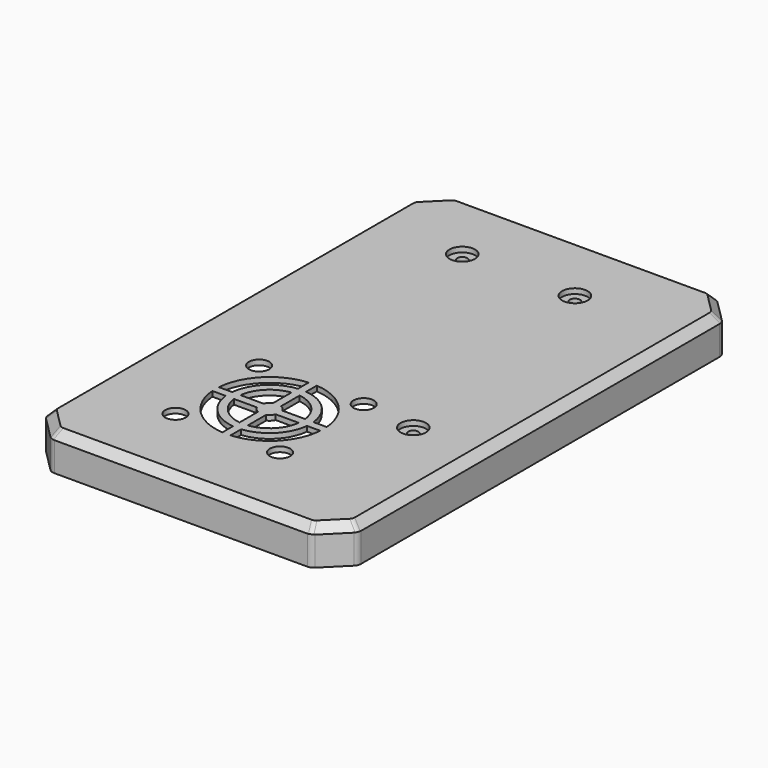
from build123d import *

# Parameters (mm, degrees)
F3_DEPTH  = 1.5875
F1_R      = 5.08
F1_R_2    = 1.5875
F4_DEPTH  = 10
F5_DEPTH  = 10
F6_R      = 3.96875
F7_DEPTH  = 1.5875
F8_R      = 3.175
F9_DEPTH  = 11.5885
F10_SIZE  = 2.54
F11_F1_R  = 2.54
F11_F2_R  = 2.54
F11_F3_R  = 2.54
F11_F4_R  = 2.54
F11_F5_R  = 2.54
F11_F6_R  = 2.54
F11_F7_R  = 2.54
F11_F8_R  = 2.54
F11_F9_R  = 2.54
F11_F10_R = 2.54
F11_F11_R = 2.54
F11_F12_R = 2.54
F11_F13_R = 2.54
F11_F14_R = 2.54
F11_F15_R = 2.54
F11_F16_R = 2.54


with BuildPart() as f3:
    # F0 (on Top) → F3 (new body)
    with BuildSketch(Plane.XY):
        Polygon((-40.4276280605, 79.0125), (-48.6375, 70.8026280605), (-48.6375, -70.8026280605), (-40.4276280605, -79.0125), (40.4276280605, -79.0125), (48.6375, -70.8026280605), (48.6375, 70.8026280605), (40.4276280605, 79.0125), align=None)
        Polygon((-45.4625, 69.4875), (-39.1125, 75.8375), (39.1125, 75.8375), (45.4625, 69.4875), (45.4625, -69.4875), (39.1125, -75.8375), (-39.1125, -75.8375), (-45.4625, -69.4875), align=None, mode=Mode.SUBTRACT)
        Polygon((39.1125, 75.8375), (-39.1125, 75.8375), (-45.4625, 69.4875), (-45.4625, -69.4875), (-39.1125, -75.8375), (39.1125, -75.8375), (45.4625, -69.4875), (45.4625, 69.4875), align=None)
    extrude(amount=F3_DEPTH)

    # F1 (on Top) → F4 (join)
    with BuildSketch(Plane.XY):
        with Locations((27.6825, -23.2224922)):
            Circle(F1_R)
        with Locations((27.6825, -23.2224922)):
            Circle(F1_R_2, mode=Mode.SUBTRACT)
        with Locations((14.9825, 55.5175)):
            Circle(F1_R)
        with Locations((14.9825, 55.5175)):
            Circle(F1_R_2, mode=Mode.SUBTRACT)
        with Locations((-20.0625, 55.5175)):
            Circle(F1_R)
        with Locations((-20.0625, 55.5175)):
            Circle(F1_R_2, mode=Mode.SUBTRACT)
    extrude(amount=-F4_DEPTH)

    # F0 (on Top) → F5 (join)
    with BuildSketch(Plane.XY):
        Polygon((-40.4276280605, 79.0125), (-48.6375, 70.8026280605), (-48.6375, -70.8026280605), (-40.4276280605, -79.0125), (40.4276280605, -79.0125), (48.6375, -70.8026280605), (48.6375, 70.8026280605), (40.4276280605, 79.0125), align=None)
        Polygon((-45.4625, 69.4875), (-39.1125, 75.8375), (39.1125, 75.8375), (45.4625, 69.4875), (45.4625, -69.4875), (39.1125, -75.8375), (-39.1125, -75.8375), (-45.4625, -69.4875), align=None, mode=Mode.SUBTRACT)
    extrude(amount=-F5_DEPTH)

    # F6 (on face) → F7 (cut)
    with BuildSketch(Plane.XY.offset(1.5875)):
        with Locations((-20.0625, 55.5175)):
            Circle(F6_R)
        with Locations((14.9825, 55.5175)):
            Circle(F6_R)
        with Locations((27.6825, -23.2224922)):
            Circle(F6_R)
    extrude(amount=-F7_DEPTH, mode=Mode.SUBTRACT)

    # F8 (on face) → F9 (cut, through all)
    with BuildSketch(Plane.XY.offset(1.5875)):
        with Locations((-22.00625, -21.06875)):
            Circle(F8_R)
        with Locations((10.5375, -21.06875)):
            Circle(F8_R)
        with Locations((10.5375, -53.6125)):
            Circle(F8_R)
        with Locations((-22.00625, -53.6125)):
            Circle(F8_R)
        with BuildLine():
            Line((-18.3707154513, -38.610625), (-22.5138820324, -38.610625))
            ThreePointArc((-22.5138820324, -38.610625), (-17.6332143604, -49.2394643604), (-7.004375, -54.1201320324))
            Line((-7.004375, -54.1201320324), (-7.004375, -49.9769654513))
            ThreePointArc((-7.004375, -49.9769654513), (-14.7146311211, -46.3208811211), (-18.3707154513, -38.610625))
        make_face()
        with BuildLine():
            ThreePointArc((-8.6443105663, -36.070625), (-7.9794390303, -35.0955609697), (-7.004375, -34.4306894337))
            Line((-7.004375, -34.4306894337), (-7.004375, -27.2603125048))
            ThreePointArc((-7.004375, -27.2603125048), (-12.9185798969, -30.1564201031), (-15.8146874952, -36.070625))
            Line((-15.8146874952, -36.070625), (-8.6443105663, -36.070625))
        make_face()
        with BuildLine():
            Line((-4.464375, -27.2603125048), (-4.464375, -34.4306894337))
            ThreePointArc((-4.464375, -34.4306894337), (-3.4893109697, -35.0955609697), (-2.8244394337, -36.070625))
            Line((-2.8244394337, -36.070625), (4.3459374952, -36.070625))
            ThreePointArc((4.3459374952, -36.070625), (1.4498298969, -30.1564201031), (-4.464375, -27.2603125048))
        make_face()
        with BuildLine():
            Line((4.3459374952, -38.610625), (-2.8244394337, -38.610625))
            ThreePointArc((-2.8244394337, -38.610625), (-3.4893109697, -39.5856890303), (-4.464375, -40.2505605663))
            Line((-4.464375, -40.2505605663), (-4.464375, -47.4209374952))
            ThreePointArc((-4.464375, -47.4209374952), (1.4498298969, -44.5248298969), (4.3459374952, -38.610625))
        make_face()
        with BuildLine():
            Line((-7.004375, -47.4209374952), (-7.004375, -40.2505605663))
            ThreePointArc((-7.004375, -40.2505605663), (-7.9794390303, -39.5856890303), (-8.6443105663, -38.610625))
            Line((-8.6443105663, -38.610625), (-15.8146874952, -38.610625))
            ThreePointArc((-15.8146874952, -38.610625), (-12.9185798969, -44.5248298969), (-7.004375, -47.4209374952))
        make_face()
        with BuildLine():
            Line((-22.5138820324, -36.070625), (-18.3707154513, -36.070625))
            ThreePointArc((-18.3707154513, -36.070625), (-14.7146311211, -28.3603688789), (-7.004375, -24.7042845487))
            Line((-7.004375, -24.7042845487), (-7.004375, -20.5611179676))
            ThreePointArc((-7.004375, -20.5611179676), (-17.6332143604, -25.4417856396), (-22.5138820324, -36.070625))
        make_face()
        with BuildLine():
            ThreePointArc((-4.464375, -24.7042845487), (3.2458811211, -28.3603688789), (6.9019654513, -36.070625))
            Line((6.9019654513, -36.070625), (11.0451320324, -36.070625))
            ThreePointArc((11.0451320324, -36.070625), (6.1644643604, -25.4417856396), (-4.464375, -20.5611179676))
            Line((-4.464375, -20.5611179676), (-4.464375, -24.7042845487))
        make_face()
        with BuildLine():
            Line((11.0451320324, -38.610625), (6.9019654513, -38.610625))
            ThreePointArc((6.9019654513, -38.610625), (3.2458811211, -46.3208811211), (-4.464375, -49.9769654513))
            Line((-4.464375, -49.9769654513), (-4.464375, -54.1201320324))
            ThreePointArc((-4.464375, -54.1201320324), (6.1644643604, -49.2394643604), (11.0451320324, -38.610625))
        make_face()
    extrude(amount=-F9_DEPTH, mode=Mode.SUBTRACT)

    # F10
    f10_edges = [f3.edges().sort_by_distance(p)[0] for p in [
        (0, 79.0125, 1.5875),
        (-44.532564, 74.907564, 1.5875),
        (-48.6375, 0, 1.5875),
        (44.532564, 74.907564, 1.5875),
        (48.6375, 0, 1.5875),
        (-44.532564, -74.907564, 1.5875),
        (0, -79.0125, 1.5875),
        (44.532564, -74.907564, 1.5875),
    ]]
    chamfer(f10_edges, length=F10_SIZE)

    # F11: fillet of radius 2.54 on 16 edges, made by hand

    # F11_f1
    f11_f1_edges = [f3.edges().sort_by_distance(p)[0] for p in [
        (-40.4276280605, 79.0125, -5.47625),
    ]]
    fillet(f11_f1_edges, radius=F11_F1_R)

    # F11_f2
    f11_f2_edges = [f3.edges().sort_by_distance(p)[0] for p in [
        (-48.6375, 70.8026280605, -5.47625),
    ]]
    fillet(f11_f2_edges, radius=F11_F2_R)

    # F11_f3
    f11_f3_edges = [f3.edges().sort_by_distance(p)[0] for p in [
        (40.4276280605, 79.0125, -5.47625),
    ]]
    fillet(f11_f3_edges, radius=F11_F3_R)

    # F11_f4
    f11_f4_edges = [f3.edges().sort_by_distance(p)[0] for p in [
        (-39.8615335712, 77.6458270063, 0.4141729937),
    ]]
    fillet(f11_f4_edges, radius=F11_F4_R)

    # F11_f5
    f11_f5_edges = [f3.edges().sort_by_distance(p)[0] for p in [
        (-47.2708270063, 70.2365335712, 0.4141729937),
    ]]
    fillet(f11_f5_edges, radius=F11_F5_R)

    # F11_f6
    f11_f6_edges = [f3.edges().sort_by_distance(p)[0] for p in [
        (-48.6375, -70.8026280605, -5.47625),
    ]]
    fillet(f11_f6_edges, radius=F11_F6_R)

    # F11_f7
    f11_f7_edges = [f3.edges().sort_by_distance(p)[0] for p in [
        (48.6375, 70.8026280605, -5.47625),
    ]]
    fillet(f11_f7_edges, radius=F11_F7_R)

    # F11_f8
    f11_f8_edges = [f3.edges().sort_by_distance(p)[0] for p in [
        (39.8615335712, 77.6458270063, 0.4141729937),
    ]]
    fillet(f11_f8_edges, radius=F11_F8_R)

    # F11_f9
    f11_f9_edges = [f3.edges().sort_by_distance(p)[0] for p in [
        (-47.2708270063, -70.2365335712, 0.4141729937),
    ]]
    fillet(f11_f9_edges, radius=F11_F9_R)

    # F11_f10
    f11_f10_edges = [f3.edges().sort_by_distance(p)[0] for p in [
        (-40.4276280605, -79.0125, -5.47625),
    ]]
    fillet(f11_f10_edges, radius=F11_F10_R)

    # F11_f11
    f11_f11_edges = [f3.edges().sort_by_distance(p)[0] for p in [
        (40.4276280605, -79.0125, -5.47625),
    ]]
    fillet(f11_f11_edges, radius=F11_F11_R)

    # F11_f12
    f11_f12_edges = [f3.edges().sort_by_distance(p)[0] for p in [
        (48.6375, -70.8026280605, -5.47625),
    ]]
    fillet(f11_f12_edges, radius=F11_F12_R)

    # F11_f13
    f11_f13_edges = [f3.edges().sort_by_distance(p)[0] for p in [
        (47.2708270063, 70.2365335712, 0.4141729937),
    ]]
    fillet(f11_f13_edges, radius=F11_F13_R)

    # F11_f14
    f11_f14_edges = [f3.edges().sort_by_distance(p)[0] for p in [
        (47.2708270063, -70.2365335712, 0.4141729937),
    ]]
    fillet(f11_f14_edges, radius=F11_F14_R)

    # F11_f15
    f11_f15_edges = [f3.edges().sort_by_distance(p)[0] for p in [
        (39.8615335712, -77.6458270063, 0.4141729937),
    ]]
    fillet(f11_f15_edges, radius=F11_F15_R)

    # F11_f16
    f11_f16_edges = [f3.edges().sort_by_distance(p)[0] for p in [
        (-39.8615335712, -77.6458270063, 0.4141729937),
    ]]
    fillet(f11_f16_edges, radius=F11_F16_R)


solid = f3.part
